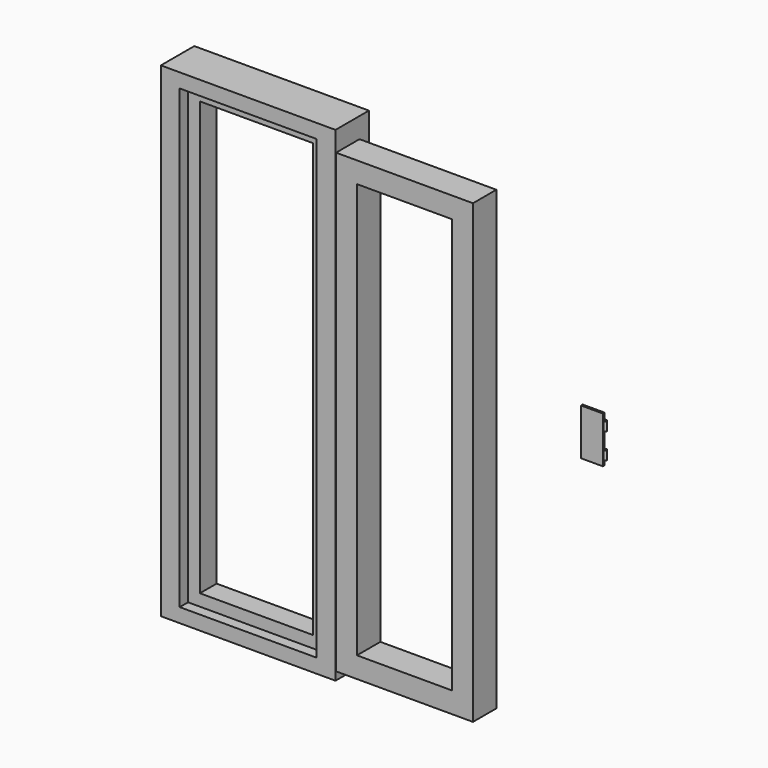
from build123d import *

# Parameters (mm, degrees)
F0_W     = 41.6117869318
F0_H     = 138.8227045536
F0_W_2   = 34.4373397529
F0_H_2   = 131.6482573748
F1_DEPTH = 3.175
F0_W_3   = 53.0909001827
F0_H_3   = 147.4320292473
F2_DEPTH = 6.35
F3_W     = 41.6117869318
F3_H     = 138.8227045536
F3_W_2   = 28.9117869318
F3_H_2   = 126.1227045536
F4_DEPTH = 8.89
F5_W     = 0.1695360988
F5_H     = 2.7262568474
F7_DEPTH = 0.3175


# Not quite as in the source:
# - a feature names something its author has since deleted; it is built from what else it names


with BuildPart() as f1:
    # F0 (on Front) → F1 (new body, symmetric)
    with BuildSketch(Plane.XZ):
        with Locations((-67.8180083632, 0)):
            Rectangle(F0_W, F0_H)
        with Locations((-67.8180083632, 0)):
            Rectangle(F0_W_2, F0_H_2, mode=Mode.SUBTRACT)
    extrude(amount=F1_DEPTH, both=True)

    # F0 (on Front) → F2 (join, symmetric)
    with BuildSketch(Plane.XZ):
        with Locations((-67.8180083632, 0)):
            Rectangle(F0_W_3, F0_H_3)
        with Locations((-67.8180083632, 0)):
            Rectangle(F0_W, F0_H, mode=Mode.SUBTRACT)
    extrude(amount=F2_DEPTH, both=True)


with BuildPart() as f4:
    # F3 (on Front) → F4 (new body)
    with BuildSketch(Plane.XZ):
        with Locations((-18.2555075735, -0.0431761146)):
            Rectangle(F3_W, F3_H)
        with Locations((-18.2555075735, -0.0431761146)):
            Rectangle(F3_W_2, F3_H_2, mode=Mode.SUBTRACT)
    extrude(amount=F4_DEPTH)


with BuildPart() as f6:
    # F5 (on Front) → F6 (revolve)
    with BuildSketch(Plane.XZ):
        with Locations((36.0232619569, 16.9993210584)):
            Rectangle(F5_W, F5_H)
    revolve(axis=Axis((35.6687009335, 0, 16.9993210584), (0, 0, -1)))


with BuildPart() as f7:
    # F5 (on Front) → F7 (new body, symmetric)
    with BuildSketch(Plane.XZ):
        Polygon((35.2293718606, 20.2041938901), (28.5136234015, 20.2041938901), (28.5136234015, 6.0779694468), (35.2293718606, 6.0779694468), (35.2293718606, 7.853361778), (35.2293718606, 10.5796186253), (35.2293718606, 15.6361926347), (35.2293718606, 18.3624494821), align=None)
    extrude(amount=F7_DEPTH, both=True)

    # F5 (on Front) → F8 (revolve)
    with BuildSketch(Plane.XZ):
        with Locations((36.0232619569, 9.2164902017)):
            Rectangle(F5_W, F5_H)
    revolve(axis=Axis((35.6687009335, 0, 9.2164902017), (0, 0, -1)))


solid = Compound([f1.part, f4.part, f6.part, f7.part])
